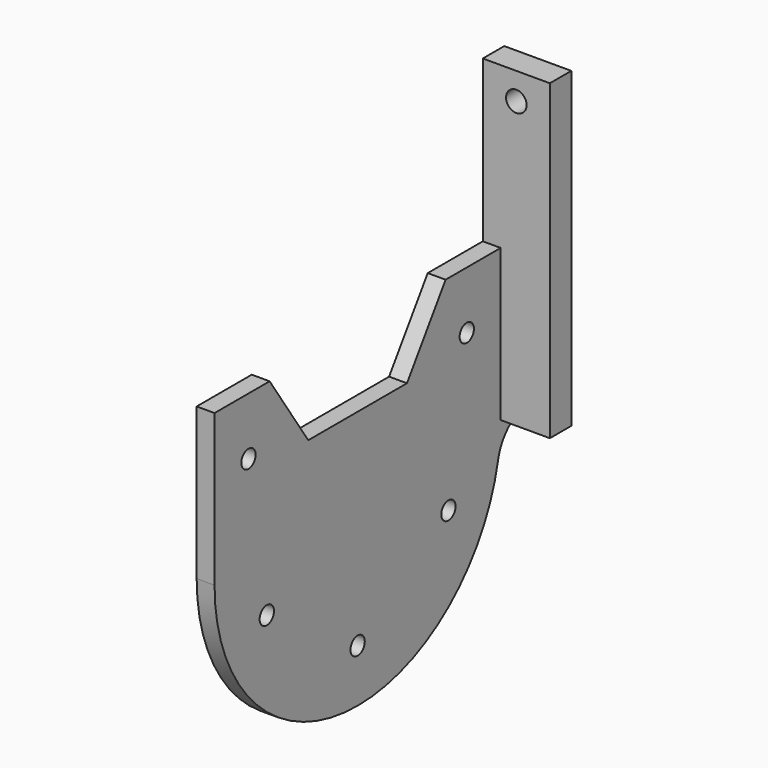
from build123d import *

# Parameters (mm, degrees)
F1_DEPTH    = 2
F2_R        = 1
F3_DEPTH    = 25
F4_R        = 1.15
F5_DEPTH    = 3
F6_T1_DEPTH = 2


# Not quite as in the source:
# - a fillet or chamfer that OpenCascade refuses, or shapes differently, is made with other operations: its cross-section is extruded or revolved along the edge and cut away or added


with BuildPart() as f1:
    # F0 (on Right) → F1 (new body)
    with BuildSketch(Plane.YZ):
        with BuildLine():
            Line((20, -8.475), (20, 8.475))
            Line((20, 8.475), (12.3, 8.475))
            Line((12.3, 8.475), (6.9, 0.475))
            Line((6.9, 0.475), (0, 0.475))
            Line((0, 0.475), (-6.9, 0.475))
            Line((-6.9, 0.475), (-12.3, 8.475))
            Line((-12.3, 8.475), (-20, 8.475))
            Line((-20, 8.475), (-20, -8.475))
            ThreePointArc((-20, -8.475), (0, -28.475), (20, -8.475))
        make_face()
    extrude(amount=F1_DEPTH)

    # F2 (on face) → F3 (cut)
    with BuildSketch(Plane.YZ.offset(2)):
        with Locations((0, -22.5554741919)):
            Circle(F2_R)
        with Locations((-12.6950368285, -14.3941175193)):
            Circle(F2_R)
        with Locations((-15.2600342408, 2.045188332)):
            Circle(F2_R)
        with Locations((12.6950368285, -14.3941175193)):
            Circle(F2_R)
        with Locations((15.2600342408, 2.045188332)):
            Circle(F2_R)
    extrude(amount=-F3_DEPTH, mode=Mode.SUBTRACT)

    # F4 (on face) → F5 (join)
    with BuildSketch(Plane(origin=(0, 20, 0), x_dir=(-1, 0, 0), z_dir=(0, 1, 0))):
        Polygon((0, 8.475), (0, 26.475), (-7.5, 26.475), (-7.5, 8.475), (-2, -8.475), (0, -8.475), align=None)
        with Locations((-3.75, 23.475)):
            Circle(F4_R, mode=Mode.SUBTRACT)
        Polygon((-2, -8.475), (-7.5, 8.475), (-7.5, -8.475), align=None)
    extrude(amount=F5_DEPTH)

    # F6: fillet of radius 5 on 1 edges, made by hand

    # F6_s2 → F6_t1 (join)
    with BuildSketch(Plane.YZ):
        with BuildLine():
            ThreePointArc((19.6347826087, -12.2796434668), (20.7982860057, -9.9181716989), (23, -8.475))
            Line((23, -8.475), (20, -8.475))
            ThreePointArc((20, -8.475), (19.9084862832, -10.3860661718), (19.6347826087, -12.2796434668))
        make_face()
    extrude(amount=F6_T1_DEPTH)


solid = f1.part
